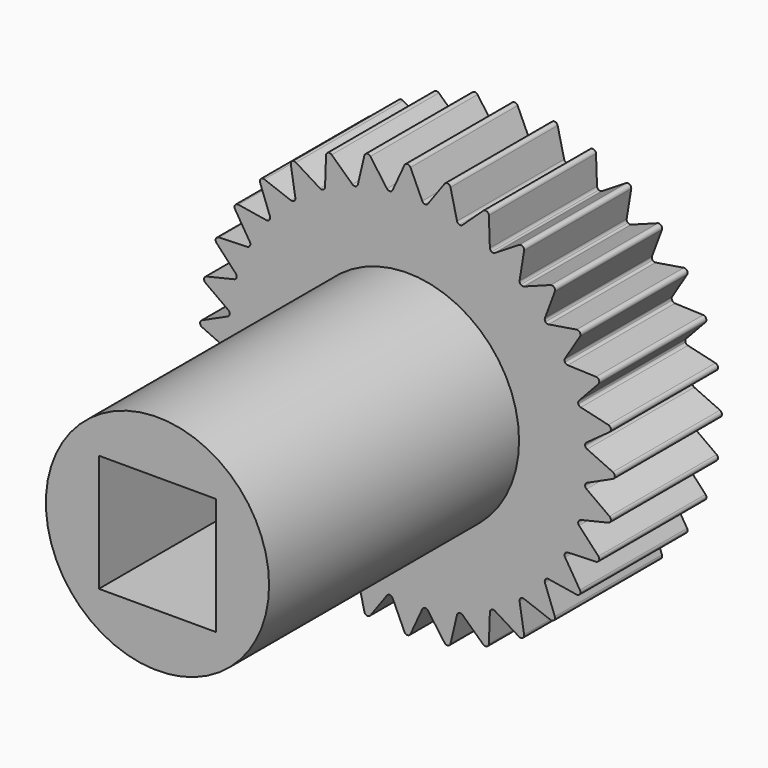
from build123d import *

# Parameters (mm, degrees)
F0_R            = 8
F0_R_2          = 5
F1_DEPTH        = 6
F2_DEPTH        = 20
F3_W            = 5.25
F3_H            = 5.25
F4_DEPTH        = 26
F6_DEPTH        = 6
F6_COPIES_COUNT = 32
F7_T1_DEPTH     = 6
F7_T3_DEPTH     = 7.6415271023


# Not quite as in the source:
# - a fillet or chamfer that OpenCascade refuses, or shapes differently, is made with other operations: its cross-section is extruded or revolved along the edge and cut away or added
# - a pattern or mirror of a feature is missing from the dataset's text; its kind, count and spacing are read off the source's solid


with BuildPart() as f1:
    # F0 (on Front) → F1 (new body)
    with BuildSketch(Plane.XZ):
        Circle(F0_R)
        Circle(F0_R_2, mode=Mode.SUBTRACT)
        Circle(F0_R_2)
    extrude(amount=F1_DEPTH)

    # F0 (on Front) → F2 (join)
    with BuildSketch(Plane.XZ):
        Circle(F0_R_2)
    extrude(amount=F2_DEPTH)

    # F3 (on face) → F4 (cut)
    with BuildSketch(Plane.XZ.offset(20)):
        Rectangle(F3_W, F3_H)
    extrude(amount=-F4_DEPTH, mode=Mode.SUBTRACT)

    # F5 (on face) → F6 (join)
    with BuildSketch(Plane(origin=(0, 0, 0), x_dir=(-1, 0, 0), z_dir=(0, 1, 0))):
        with BuildLine():
            ThreePointArc((-0.6993297572, 7.969375), (-0.35, 7.9923400829), (0, 8))
            ThreePointArc((0, 8), (0.35, 7.9923400829), (0.6993297572, 7.969375))
            Line((0.6993297572, 7.969375), (0, 9.5))
            Line((0, 9.5), (-0.6993297572, 7.969375))
        make_face()
    f6 = extrude(amount=-F6_DEPTH)

    # F6_copies: F6 ×32 about axis
    f6_copies_axis = Axis((0, 0, 0), (0, 1, 0))
    for i in range(1, F6_COPIES_COUNT):
        add(f6.rotate(f6_copies_axis, i * 360 / F6_COPIES_COUNT))

    # F7: fillet of radius 0.15 on 96 edges, made by hand

    # F7_s2 → F7_t1 (join)
    with BuildSketch(Plane.XZ):
        with BuildLine():
            ThreePointArc((0.6632529517, 8.0483364054), (0.7125009612, 7.9886122754), (0.7849689133, 7.9613958453))
            ThreePointArc((0.7849689133, 7.9613958453), (0.7421600586, 7.9655005146), (0.6993297572, 7.969375))
            Line((0.6993297572, 7.969375), (0.6632529517, 8.0483364054))
        make_face()
        with BuildLine():
            ThreePointArc((-0.7849689133, 7.9613958453), (-0.7125009612, 7.9886122754), (-0.6632529517, 8.0483364054))
            Line((-0.6632529517, 8.0483364054), (-0.6993297572, 7.969375))
            ThreePointArc((-0.6993297572, 7.969375), (-0.7421600586, 7.9655005146), (-0.7849689133, 7.9613958453))
        make_face()
        with BuildLine():
            ThreePointArc((-0.7833053234, 7.9615596946), (-0.8596904862, 7.9741153725), (-0.9196438088, 8.0230841101))
            Line((-0.9196438088, 8.0230841101), (-0.868855603, 7.9526781616))
            ThreePointArc((-0.868855603, 7.9526781616), (-0.8260923992, 7.9572339005), (-0.7833053234, 7.9615596946))
        make_face()
        with BuildLine():
            ThreePointArc((-2.3214775758, 7.6557652697), (-2.3988445104, 7.6531776878), (-2.4671991735, 7.6895091918))
            Line((-2.4671991735, 7.6895091918), (-2.4036513296, 7.6303643613))
            ThreePointArc((-2.4036513296, 7.6303643613), (-2.3625985894, 7.6431752502), (-2.3214775758, 7.6557652697))
        make_face()
        with BuildLine():
            ThreePointArc((-2.3230772349, 7.6552800184), (-2.2573113963, 7.6961112886), (-2.2206612733, 7.7642956462))
            Line((-2.2206612733, 7.7642956462), (-2.2406402671, 7.6798132265))
            ThreePointArc((-2.2406402671, 7.6798132265), (-2.2818917216, 7.6676574109), (-2.3230772349, 7.6552800184))
        make_face()
        with BuildLine():
            ThreePointArc((-3.6927308274, 7.1818773596), (-3.7153746204, 7.107853061), (-3.7719110012, 7.0549760736))
            ThreePointArc((-3.7719110012, 7.0549760736), (-3.7339315654, 7.075150533), (-3.695844228, 7.0951205375))
            Line((-3.695844228, 7.0951205375), (-3.6927308274, 7.1818773596))
        make_face()
        with BuildLine():
            ThreePointArc((-3.7704367469, 7.0557640789), (-3.8458122853, 7.0381326765), (-3.9199414575, 7.0604307476))
            Line((-3.9199414575, 7.0604307476), (-3.8460760836, 7.0148199377))
            ThreePointArc((-3.8460760836, 7.0148199377), (-3.8083114408, 7.0353936613), (-3.7704367469, 7.0557640789))
        make_face()
        with BuildLine():
            ThreePointArc((-5.0228908068, 6.3234635537), (-5.0306580813, 6.2464440264), (-5.0757923429, 6.1835533548))
            ThreePointArc((-5.0757923429, 6.1835533548), (-5.0424785132, 6.2107495879), (-5.0090189679, 6.2377663454))
            Line((-5.0090189679, 6.2377663454), (-5.0228908068, 6.3234635537))
        make_face()
        with BuildLine():
            ThreePointArc((-5.0745001483, 6.1846138315), (-5.1449876509, 6.1526161735), (-5.2220425897, 6.1600239093))
            Line((-5.2220425897, 6.1600239093), (-5.1406982907, 6.129699918))
            ThreePointArc((-5.1406982907, 6.129699918), (-5.1076730192, 6.1572458396), (-5.0745001483, 6.1846138315))
        make_face()
        with BuildLine():
            ThreePointArc((-6.1600239093, 5.2220425897), (-6.1526161735, 5.1449876509), (-6.1846138315, 5.0745001483))
            ThreePointArc((-6.1846138315, 5.0745001483), (-6.1572458396, 5.1076730192), (-6.129699918, 5.1406982907))
            Line((-6.129699918, 5.1406982907), (-6.1600239093, 5.2220425897))
        make_face()
        with BuildLine():
            ThreePointArc((-6.1835533548, 5.0757923429), (-6.2464440264, 5.0306580813), (-6.3234635537, 5.0228908068))
            Line((-6.3234635537, 5.0228908068), (-6.2377663454, 5.0090189679))
            ThreePointArc((-6.2377663454, 5.0090189679), (-6.2107495879, 5.0424785132), (-6.1835533548, 5.0757923429))
        make_face()
        with BuildLine():
            ThreePointArc((-7.0604307476, 3.9199414575), (-7.0381326765, 3.8458122853), (-7.0557640789, 3.7704367469))
            ThreePointArc((-7.0557640789, 3.7704367469), (-7.0353936613, 3.8083114408), (-7.0148199377, 3.8460760836))
            Line((-7.0148199377, 3.8460760836), (-7.0604307476, 3.9199414575))
        make_face()
        with BuildLine():
            ThreePointArc((-7.0549760736, 3.7719110012), (-7.107853061, 3.7153746204), (-7.1818773596, 3.6927308274))
            Line((-7.1818773596, 3.6927308274), (-7.0951205375, 3.695844228))
            ThreePointArc((-7.0951205375, 3.695844228), (-7.075150533, 3.7339315654), (-7.0549760736, 3.7719110012))
        make_face()
        with BuildLine():
            ThreePointArc((-7.6895091918, 2.4671991735), (-7.6531776878, 2.3988445104), (-7.6557652697, 2.3214775758))
            ThreePointArc((-7.6557652697, 2.3214775758), (-7.6431752502, 2.3625985894), (-7.6303643613, 2.4036513296))
            Line((-7.6303643613, 2.4036513296), (-7.6895091918, 2.4671991735))
        make_face()
        with BuildLine():
            ThreePointArc((-7.6552800184, 2.3230772349), (-7.6961112886, 2.2573113963), (-7.7642956462, 2.2206612733))
            Line((-7.7642956462, 2.2206612733), (-7.6798132265, 2.2406402671))
            ThreePointArc((-7.6798132265, 2.2406402671), (-7.6676574109, 2.2818917216), (-7.6552800184, 2.3230772349))
        make_face()
        with BuildLine():
            ThreePointArc((-8.0230841101, 0.9196438088), (-7.9741153725, 0.8596904862), (-7.9615596946, 0.7833053234))
            ThreePointArc((-7.9615596946, 0.7833053234), (-7.9572339005, 0.8260923992), (-7.9526781616, 0.868855603))
            Line((-7.9526781616, 0.868855603), (-8.0230841101, 0.9196438088))
        make_face()
        with BuildLine():
            ThreePointArc((-7.9613958453, 0.7849689133), (-7.9886122754, 0.7125009612), (-8.0483364054, 0.6632529517))
            Line((-8.0483364054, 0.6632529517), (-7.969375, 0.6993297572))
            ThreePointArc((-7.969375, 0.6993297572), (-7.9655005146, 0.7421600586), (-7.9613958453, 0.7849689133))
        make_face()
        with BuildLine():
            ThreePointArc((-8.0483364054, -0.6632529517), (-7.9886122754, -0.7125009612), (-7.9613958453, -0.7849689133))
            ThreePointArc((-7.9613958453, -0.7849689133), (-7.9655005146, -0.7421600586), (-7.969375, -0.6993297572))
            Line((-7.969375, -0.6993297572), (-8.0483364054, -0.6632529517))
        make_face()
        with BuildLine():
            ThreePointArc((-7.9615596946, -0.7833053234), (-7.9741153725, -0.8596904862), (-8.0230841101, -0.9196438088))
            Line((-8.0230841101, -0.9196438088), (-7.9526781616, -0.868855603))
            ThreePointArc((-7.9526781616, -0.868855603), (-7.9572339005, -0.8260923992), (-7.9615596946, -0.7833053234))
        make_face()
        with BuildLine():
            ThreePointArc((-7.7642956462, -2.2206612733), (-7.6961112886, -2.2573113963), (-7.6552800184, -2.3230772349))
            ThreePointArc((-7.6552800184, -2.3230772349), (-7.6676574109, -2.2818917216), (-7.6798132265, -2.2406402671))
            Line((-7.6798132265, -2.2406402671), (-7.7642956462, -2.2206612733))
        make_face()
        with BuildLine():
            ThreePointArc((-7.6557652697, -2.3214775758), (-7.6531776878, -2.3988445104), (-7.6895091918, -2.4671991735))
            Line((-7.6895091918, -2.4671991735), (-7.6303643613, -2.4036513296))
            ThreePointArc((-7.6303643613, -2.4036513296), (-7.6431752502, -2.3625985894), (-7.6557652697, -2.3214775758))
        make_face()
        with BuildLine():
            ThreePointArc((-7.1818773596, -3.6927308274), (-7.107853061, -3.7153746204), (-7.0549760736, -3.7719110012))
            ThreePointArc((-7.0549760736, -3.7719110012), (-7.075150533, -3.7339315654), (-7.0951205375, -3.695844228))
            Line((-7.0951205375, -3.695844228), (-7.1818773596, -3.6927308274))
        make_face()
        with BuildLine():
            ThreePointArc((-7.0557640789, -3.7704367469), (-7.0381326765, -3.8458122853), (-7.0604307476, -3.9199414575))
            Line((-7.0604307476, -3.9199414575), (-7.0148199377, -3.8460760836))
            ThreePointArc((-7.0148199377, -3.8460760836), (-7.0353936613, -3.8083114408), (-7.0557640789, -3.7704367469))
        make_face()
        with BuildLine():
            ThreePointArc((-6.3234635537, -5.0228908068), (-6.2464440264, -5.0306580813), (-6.1835533548, -5.0757923429))
            ThreePointArc((-6.1835533548, -5.0757923429), (-6.2107495879, -5.0424785132), (-6.2377663454, -5.0090189679))
            Line((-6.2377663454, -5.0090189679), (-6.3234635537, -5.0228908068))
        make_face()
        with BuildLine():
            ThreePointArc((-6.1846138315, -5.0745001483), (-6.1526161735, -5.1449876509), (-6.1600239093, -5.2220425897))
            Line((-6.1600239093, -5.2220425897), (-6.129699918, -5.1406982907))
            ThreePointArc((-6.129699918, -5.1406982907), (-6.1572458396, -5.1076730192), (-6.1846138315, -5.0745001483))
        make_face()
        with BuildLine():
            ThreePointArc((-5.2220425897, -6.1600239093), (-5.1449876509, -6.1526161735), (-5.0745001483, -6.1846138315))
            ThreePointArc((-5.0745001483, -6.1846138315), (-5.1076730192, -6.1572458396), (-5.1406982907, -6.129699918))
            Line((-5.1406982907, -6.129699918), (-5.2220425897, -6.1600239093))
        make_face()
        with BuildLine():
            ThreePointArc((-5.0757923429, -6.1835533548), (-5.0306580813, -6.2464440264), (-5.0228908068, -6.3234635537))
            Line((-5.0228908068, -6.3234635537), (-5.0090189679, -6.2377663454))
            ThreePointArc((-5.0090189679, -6.2377663454), (-5.0424785132, -6.2107495879), (-5.0757923429, -6.1835533548))
        make_face()
        with BuildLine():
            ThreePointArc((-3.9199414575, -7.0604307476), (-3.8458122853, -7.0381326765), (-3.7704367469, -7.0557640789))
            ThreePointArc((-3.7704367469, -7.0557640789), (-3.8083114408, -7.0353936613), (-3.8460760836, -7.0148199377))
            Line((-3.8460760836, -7.0148199377), (-3.9199414575, -7.0604307476))
        make_face()
        with BuildLine():
            ThreePointArc((-3.7719110012, -7.0549760736), (-3.7153746204, -7.107853061), (-3.6927308274, -7.1818773596))
            Line((-3.6927308274, -7.1818773596), (-3.695844228, -7.0951205375))
            ThreePointArc((-3.695844228, -7.0951205375), (-3.7339315654, -7.075150533), (-3.7719110012, -7.0549760736))
        make_face()
        with BuildLine():
            ThreePointArc((-2.4671991735, -7.6895091918), (-2.3988445104, -7.6531776878), (-2.3214775758, -7.6557652697))
            ThreePointArc((-2.3214775758, -7.6557652697), (-2.3625985894, -7.6431752502), (-2.4036513296, -7.6303643613))
            Line((-2.4036513296, -7.6303643613), (-2.4671991735, -7.6895091918))
        make_face()
        with BuildLine():
            ThreePointArc((-2.3230772349, -7.6552800184), (-2.2573113963, -7.6961112886), (-2.2206612733, -7.7642956462))
            Line((-2.2206612733, -7.7642956462), (-2.2406402671, -7.6798132265))
            ThreePointArc((-2.2406402671, -7.6798132265), (-2.2818917216, -7.6676574109), (-2.3230772349, -7.6552800184))
        make_face()
        with BuildLine():
            ThreePointArc((-0.9196438088, -8.0230841101), (-0.8596904862, -7.9741153725), (-0.7833053234, -7.9615596946))
            ThreePointArc((-0.7833053234, -7.9615596946), (-0.8260923992, -7.9572339005), (-0.868855603, -7.9526781616))
            Line((-0.868855603, -7.9526781616), (-0.9196438088, -8.0230841101))
        make_face()
        with BuildLine():
            ThreePointArc((-0.7849689133, -7.9613958453), (-0.7125009612, -7.9886122754), (-0.6632529517, -8.0483364054))
            Line((-0.6632529517, -8.0483364054), (-0.6993297572, -7.969375))
            ThreePointArc((-0.6993297572, -7.969375), (-0.7421600586, -7.9655005146), (-0.7849689133, -7.9613958453))
        make_face()
        with BuildLine():
            ThreePointArc((0.6632529517, -8.0483364054), (0.7125009612, -7.9886122754), (0.7849689133, -7.9613958453))
            ThreePointArc((0.7849689133, -7.9613958453), (0.7421600586, -7.9655005146), (0.6993297572, -7.969375))
            Line((0.6993297572, -7.969375), (0.6632529517, -8.0483364054))
        make_face()
        with BuildLine():
            ThreePointArc((0.7833053234, -7.9615596946), (0.8596904862, -7.9741153725), (0.9196438088, -8.0230841101))
            Line((0.9196438088, -8.0230841101), (0.868855603, -7.9526781616))
            ThreePointArc((0.868855603, -7.9526781616), (0.8260923992, -7.9572339005), (0.7833053234, -7.9615596946))
        make_face()
        with BuildLine():
            ThreePointArc((2.2206612733, -7.7642956462), (2.2573113963, -7.6961112886), (2.3230772349, -7.6552800184))
            ThreePointArc((2.3230772349, -7.6552800184), (2.2818917216, -7.6676574109), (2.2406402671, -7.6798132265))
            Line((2.2406402671, -7.6798132265), (2.2206612733, -7.7642956462))
        make_face()
        with BuildLine():
            ThreePointArc((2.3214775758, -7.6557652697), (2.3988445104, -7.6531776878), (2.4671991735, -7.6895091918))
            Line((2.4671991735, -7.6895091918), (2.4036513296, -7.6303643613))
            ThreePointArc((2.4036513296, -7.6303643613), (2.3625985894, -7.6431752502), (2.3214775758, -7.6557652697))
        make_face()
        with BuildLine():
            ThreePointArc((3.6927308274, -7.1818773596), (3.7153746204, -7.107853061), (3.7719110012, -7.0549760736))
            ThreePointArc((3.7719110012, -7.0549760736), (3.7339315654, -7.075150533), (3.695844228, -7.0951205375))
            Line((3.695844228, -7.0951205375), (3.6927308274, -7.1818773596))
        make_face()
        with BuildLine():
            ThreePointArc((3.7704367469, -7.0557640789), (3.8458122853, -7.0381326765), (3.9199414575, -7.0604307476))
            Line((3.9199414575, -7.0604307476), (3.8460760836, -7.0148199377))
            ThreePointArc((3.8460760836, -7.0148199377), (3.8083114408, -7.0353936613), (3.7704367469, -7.0557640789))
        make_face()
        with BuildLine():
            ThreePointArc((5.0228908068, -6.3234635537), (5.0306580813, -6.2464440264), (5.0757923429, -6.1835533548))
            ThreePointArc((5.0757923429, -6.1835533548), (5.0424785132, -6.2107495879), (5.0090189679, -6.2377663454))
            Line((5.0090189679, -6.2377663454), (5.0228908068, -6.3234635537))
        make_face()
        with BuildLine():
            ThreePointArc((5.0745001483, -6.1846138315), (5.1449876509, -6.1526161735), (5.2220425897, -6.1600239093))
            Line((5.2220425897, -6.1600239093), (5.1406982907, -6.129699918))
            ThreePointArc((5.1406982907, -6.129699918), (5.1076730192, -6.1572458396), (5.0745001483, -6.1846138315))
        make_face()
        with BuildLine():
            ThreePointArc((6.1600239093, -5.2220425897), (6.1526161735, -5.1449876509), (6.1846138315, -5.0745001483))
            ThreePointArc((6.1846138315, -5.0745001483), (6.1572458396, -5.1076730192), (6.129699918, -5.1406982907))
            Line((6.129699918, -5.1406982907), (6.1600239093, -5.2220425897))
        make_face()
        with BuildLine():
            ThreePointArc((6.1835533548, -5.0757923429), (6.2464440264, -5.0306580813), (6.3234635537, -5.0228908068))
            Line((6.3234635537, -5.0228908068), (6.2377663454, -5.0090189679))
            ThreePointArc((6.2377663454, -5.0090189679), (6.2107495879, -5.0424785132), (6.1835533548, -5.0757923429))
        make_face()
        with BuildLine():
            ThreePointArc((7.0604307476, -3.9199414575), (7.0381326765, -3.8458122853), (7.0557640789, -3.7704367469))
            ThreePointArc((7.0557640789, -3.7704367469), (7.0353936613, -3.8083114408), (7.0148199377, -3.8460760836))
            Line((7.0148199377, -3.8460760836), (7.0604307476, -3.9199414575))
        make_face()
        with BuildLine():
            ThreePointArc((7.0549760736, -3.7719110012), (7.107853061, -3.7153746204), (7.1818773596, -3.6927308274))
            Line((7.1818773596, -3.6927308274), (7.0951205375, -3.695844228))
            ThreePointArc((7.0951205375, -3.695844228), (7.075150533, -3.7339315654), (7.0549760736, -3.7719110012))
        make_face()
        with BuildLine():
            ThreePointArc((7.6895091918, -2.4671991735), (7.6531776878, -2.3988445104), (7.6557652697, -2.3214775758))
            ThreePointArc((7.6557652697, -2.3214775758), (7.6431752502, -2.3625985894), (7.6303643613, -2.4036513296))
            Line((7.6303643613, -2.4036513296), (7.6895091918, -2.4671991735))
        make_face()
        with BuildLine():
            ThreePointArc((7.6552800184, -2.3230772349), (7.6961112886, -2.2573113963), (7.7642956462, -2.2206612733))
            Line((7.7642956462, -2.2206612733), (7.6798132265, -2.2406402671))
            ThreePointArc((7.6798132265, -2.2406402671), (7.6676574109, -2.2818917216), (7.6552800184, -2.3230772349))
        make_face()
        with BuildLine():
            ThreePointArc((8.0230841101, -0.9196438088), (7.9741153725, -0.8596904862), (7.9615596946, -0.7833053234))
            ThreePointArc((7.9615596946, -0.7833053234), (7.9572339005, -0.8260923992), (7.9526781616, -0.868855603))
            Line((7.9526781616, -0.868855603), (8.0230841101, -0.9196438088))
        make_face()
        with BuildLine():
            ThreePointArc((7.9613958453, -0.7849689133), (7.9886122754, -0.7125009612), (8.0483364054, -0.6632529517))
            Line((8.0483364054, -0.6632529517), (7.969375, -0.6993297572))
            ThreePointArc((7.969375, -0.6993297572), (7.9655005146, -0.7421600586), (7.9613958453, -0.7849689133))
        make_face()
        with BuildLine():
            ThreePointArc((8.0483364054, 0.6632529517), (7.9886122754, 0.7125009612), (7.9613958453, 0.7849689133))
            ThreePointArc((7.9613958453, 0.7849689133), (7.9655005146, 0.7421600586), (7.969375, 0.6993297572))
            Line((7.969375, 0.6993297572), (8.0483364054, 0.6632529517))
        make_face()
        with BuildLine():
            ThreePointArc((7.9615596946, 0.7833053234), (7.9741153725, 0.8596904862), (8.0230841101, 0.9196438088))
            Line((8.0230841101, 0.9196438088), (7.9526781616, 0.868855603))
            ThreePointArc((7.9526781616, 0.868855603), (7.9572339005, 0.8260923992), (7.9615596946, 0.7833053234))
        make_face()
        with BuildLine():
            ThreePointArc((7.7642956462, 2.2206612733), (7.6961112886, 2.2573113963), (7.6552800184, 2.3230772349))
            ThreePointArc((7.6552800184, 2.3230772349), (7.6676574109, 2.2818917216), (7.6798132265, 2.2406402671))
            Line((7.6798132265, 2.2406402671), (7.7642956462, 2.2206612733))
        make_face()
        with BuildLine():
            ThreePointArc((7.6557652697, 2.3214775758), (7.6531776878, 2.3988445104), (7.6895091918, 2.4671991735))
            Line((7.6895091918, 2.4671991735), (7.6303643613, 2.4036513296))
            ThreePointArc((7.6303643613, 2.4036513296), (7.6431752502, 2.3625985894), (7.6557652697, 2.3214775758))
        make_face()
        with BuildLine():
            ThreePointArc((7.1818773596, 3.6927308274), (7.107853061, 3.7153746204), (7.0549760736, 3.7719110012))
            ThreePointArc((7.0549760736, 3.7719110012), (7.075150533, 3.7339315654), (7.0951205375, 3.695844228))
            Line((7.0951205375, 3.695844228), (7.1818773596, 3.6927308274))
        make_face()
        with BuildLine():
            ThreePointArc((7.0557640789, 3.7704367469), (7.0381326765, 3.8458122853), (7.0604307476, 3.9199414575))
            Line((7.0604307476, 3.9199414575), (7.0148199377, 3.8460760836))
            ThreePointArc((7.0148199377, 3.8460760836), (7.0353936613, 3.8083114408), (7.0557640789, 3.7704367469))
        make_face()
        with BuildLine():
            ThreePointArc((6.3234635537, 5.0228908068), (6.2464440264, 5.0306580813), (6.1835533548, 5.0757923429))
            ThreePointArc((6.1835533548, 5.0757923429), (6.2107495879, 5.0424785132), (6.2377663454, 5.0090189679))
            Line((6.2377663454, 5.0090189679), (6.3234635537, 5.0228908068))
        make_face()
        with BuildLine():
            ThreePointArc((6.1846138315, 5.0745001483), (6.1526161735, 5.1449876509), (6.1600239093, 5.2220425897))
            Line((6.1600239093, 5.2220425897), (6.129699918, 5.1406982907))
            ThreePointArc((6.129699918, 5.1406982907), (6.1572458396, 5.1076730192), (6.1846138315, 5.0745001483))
        make_face()
        with BuildLine():
            ThreePointArc((5.2220425897, 6.1600239093), (5.1449876509, 6.1526161735), (5.0745001483, 6.1846138315))
            ThreePointArc((5.0745001483, 6.1846138315), (5.1076730192, 6.1572458396), (5.1406982907, 6.129699918))
            Line((5.1406982907, 6.129699918), (5.2220425897, 6.1600239093))
        make_face()
        with BuildLine():
            ThreePointArc((5.0757923429, 6.1835533548), (5.0306580813, 6.2464440264), (5.0228908068, 6.3234635537))
            Line((5.0228908068, 6.3234635537), (5.0090189679, 6.2377663454))
            ThreePointArc((5.0090189679, 6.2377663454), (5.0424785132, 6.2107495879), (5.0757923429, 6.1835533548))
        make_face()
        with BuildLine():
            ThreePointArc((3.9199414575, 7.0604307476), (3.8458122853, 7.0381326765), (3.7704367469, 7.0557640789))
            ThreePointArc((3.7704367469, 7.0557640789), (3.8083114408, 7.0353936613), (3.8460760836, 7.0148199377))
            Line((3.8460760836, 7.0148199377), (3.9199414575, 7.0604307476))
        make_face()
        with BuildLine():
            ThreePointArc((3.7719110012, 7.0549760736), (3.7153746204, 7.107853061), (3.6927308274, 7.1818773596))
            Line((3.6927308274, 7.1818773596), (3.695844228, 7.0951205375))
            ThreePointArc((3.695844228, 7.0951205375), (3.7339315654, 7.075150533), (3.7719110012, 7.0549760736))
        make_face()
        with BuildLine():
            ThreePointArc((2.4671991735, 7.6895091918), (2.3988445104, 7.6531776878), (2.3214775758, 7.6557652697))
            ThreePointArc((2.3214775758, 7.6557652697), (2.3625985894, 7.6431752502), (2.4036513296, 7.6303643613))
            Line((2.4036513296, 7.6303643613), (2.4671991735, 7.6895091918))
        make_face()
        with BuildLine():
            ThreePointArc((2.3230772349, 7.6552800184), (2.2573113963, 7.6961112886), (2.2206612733, 7.7642956462))
            Line((2.2206612733, 7.7642956462), (2.2406402671, 7.6798132265))
            ThreePointArc((2.2406402671, 7.6798132265), (2.2818917216, 7.6676574109), (2.3230772349, 7.6552800184))
        make_face()
        with BuildLine():
            ThreePointArc((0.9196438088, 8.0230841101), (0.8596904862, 7.9741153725), (0.7833053234, 7.9615596946))
            ThreePointArc((0.7833053234, 7.9615596946), (0.8260923992, 7.9572339005), (0.868855603, 7.9526781616))
            Line((0.868855603, 7.9526781616), (0.9196438088, 8.0230841101))
        make_face()
    extrude(amount=F7_T1_DEPTH)

    # F7_s4 → F7_t3 (cut)
    with BuildSketch(Plane.XZ.offset(-0.8207635512)):
        with BuildLine():
            ThreePointArc((0.1364341287, 9.20138624), (0, 9.2890506281), (-0.1364341287, 9.20138624))
            Line((-0.1364341287, 9.20138624), (0, 9.5))
            Line((0, 9.5), (0.1364341287, 9.20138624))
        make_face()
        with BuildLine():
            ThreePointArc((-1.6612888194, 9.0512011616), (-1.8122038783, 9.1105641249), (-1.9289139898, 8.9979672054))
            Line((-1.9289139898, 8.9979672054), (-1.8533580592, 9.3174601638))
            Line((-1.8533580592, 9.3174601638), (-1.6612888194, 9.0512011616))
        make_face()
        with BuildLine():
            ThreePointArc((-3.3951693698, 8.5531834986), (-3.5547657778, 8.5819637517), (-3.6472667679, 8.4487613372))
            Line((-3.6472667679, 8.4487613372), (-3.6354926075, 8.7768555589))
            Line((-3.6354926075, 8.7768555589), (-3.3951693698, 8.5531834986))
        make_face()
        with BuildLine():
            ThreePointArc((-4.9985754654, 7.7264717903), (-5.160720022, 7.7235633244), (-5.2254571296, 7.574874309))
            Line((-5.2254571296, 7.574874309), (-5.2779172137, 7.8989613169))
            Line((-5.2779172137, 7.8989613169), (-4.9985754654, 7.7264717903))
        make_face()
        with BuildLine():
            ThreePointArc((-6.4098891091, 6.6028361043), (-6.5683506899, 6.5683506899), (-6.6028361043, 6.4098891091))
            Line((-6.6028361043, 6.4098891091), (-6.7175144213, 6.7175144213))
            Line((-6.7175144213, 6.7175144213), (-6.4098891091, 6.6028361043))
        make_face()
        with BuildLine():
            ThreePointArc((-7.574874309, 5.2254571296), (-7.7235633244, 5.160720022), (-7.7264717903, 4.9985754654))
            Line((-7.7264717903, 4.9985754654), (-7.8989613169, 5.2779172137))
            Line((-7.8989613169, 5.2779172137), (-7.574874309, 5.2254571296))
        make_face()
        with BuildLine():
            ThreePointArc((-8.4487613372, 3.6472667679), (-8.5819637517, 3.5547657778), (-8.5531834986, 3.3951693698))
            Line((-8.5531834986, 3.3951693698), (-8.7768555589, 3.6354926075))
            Line((-8.7768555589, 3.6354926075), (-8.4487613372, 3.6472667679))
        make_face()
        with BuildLine():
            ThreePointArc((-8.9979672054, 1.9289139898), (-9.1105641249, 1.8122038783), (-9.0512011616, 1.6612888194))
            Line((-9.0512011616, 1.6612888194), (-9.3174601638, 1.8533580592))
            Line((-9.3174601638, 1.8533580592), (-8.9979672054, 1.9289139898))
        make_face()
        with BuildLine():
            ThreePointArc((-9.20138624, 0.1364341287), (-9.2890506281, 0), (-9.20138624, -0.1364341287))
            Line((-9.20138624, -0.1364341287), (-9.5, 0))
            Line((-9.5, 0), (-9.20138624, 0.1364341287))
        make_face()
        with BuildLine():
            ThreePointArc((-9.0512011616, -1.6612888194), (-9.1105641249, -1.8122038783), (-8.9979672054, -1.9289139898))
            Line((-8.9979672054, -1.9289139898), (-9.3174601638, -1.8533580592))
            Line((-9.3174601638, -1.8533580592), (-9.0512011616, -1.6612888194))
        make_face()
        with BuildLine():
            ThreePointArc((-8.5531834986, -3.3951693698), (-8.5819637517, -3.5547657778), (-8.4487613372, -3.6472667679))
            Line((-8.4487613372, -3.6472667679), (-8.7768555589, -3.6354926075))
            Line((-8.7768555589, -3.6354926075), (-8.5531834986, -3.3951693698))
        make_face()
        with BuildLine():
            ThreePointArc((-7.7264717903, -4.9985754654), (-7.7235633244, -5.160720022), (-7.574874309, -5.2254571296))
            Line((-7.574874309, -5.2254571296), (-7.8989613169, -5.2779172137))
            Line((-7.8989613169, -5.2779172137), (-7.7264717903, -4.9985754654))
        make_face()
        with BuildLine():
            ThreePointArc((-6.6028361043, -6.4098891091), (-6.5683506899, -6.5683506899), (-6.4098891091, -6.6028361043))
            Line((-6.4098891091, -6.6028361043), (-6.7175144213, -6.7175144213))
            Line((-6.7175144213, -6.7175144213), (-6.6028361043, -6.4098891091))
        make_face()
        with BuildLine():
            ThreePointArc((-5.2254571296, -7.574874309), (-5.160720022, -7.7235633244), (-4.9985754654, -7.7264717903))
            Line((-4.9985754654, -7.7264717903), (-5.2779172137, -7.8989613169))
            Line((-5.2779172137, -7.8989613169), (-5.2254571296, -7.574874309))
        make_face()
        with BuildLine():
            ThreePointArc((-3.6472667679, -8.4487613372), (-3.5547657778, -8.5819637517), (-3.3951693698, -8.5531834986))
            Line((-3.3951693698, -8.5531834986), (-3.6354926075, -8.7768555589))
            Line((-3.6354926075, -8.7768555589), (-3.6472667679, -8.4487613372))
        make_face()
        with BuildLine():
            ThreePointArc((-1.9289139898, -8.9979672054), (-1.8122038783, -9.1105641249), (-1.6612888194, -9.0512011616))
            Line((-1.6612888194, -9.0512011616), (-1.8533580592, -9.3174601638))
            Line((-1.8533580592, -9.3174601638), (-1.9289139898, -8.9979672054))
        make_face()
        with BuildLine():
            ThreePointArc((-0.1364341287, -9.20138624), (0, -9.2890506281), (0.1364341287, -9.20138624))
            Line((0.1364341287, -9.20138624), (0, -9.5))
            Line((0, -9.5), (-0.1364341287, -9.20138624))
        make_face()
        with BuildLine():
            ThreePointArc((1.6612888194, -9.0512011616), (1.8122038783, -9.1105641249), (1.9289139898, -8.9979672054))
            Line((1.9289139898, -8.9979672054), (1.8533580592, -9.3174601638))
            Line((1.8533580592, -9.3174601638), (1.6612888194, -9.0512011616))
        make_face()
        with BuildLine():
            ThreePointArc((3.3951693698, -8.5531834986), (3.5547657778, -8.5819637517), (3.6472667679, -8.4487613372))
            Line((3.6472667679, -8.4487613372), (3.6354926075, -8.7768555589))
            Line((3.6354926075, -8.7768555589), (3.3951693698, -8.5531834986))
        make_face()
        with BuildLine():
            ThreePointArc((4.9985754654, -7.7264717903), (5.160720022, -7.7235633244), (5.2254571296, -7.574874309))
            Line((5.2254571296, -7.574874309), (5.2779172137, -7.8989613169))
            Line((5.2779172137, -7.8989613169), (4.9985754654, -7.7264717903))
        make_face()
        with BuildLine():
            ThreePointArc((6.4098891091, -6.6028361043), (6.5683506899, -6.5683506899), (6.6028361043, -6.4098891091))
            Line((6.6028361043, -6.4098891091), (6.7175144213, -6.7175144213))
            Line((6.7175144213, -6.7175144213), (6.4098891091, -6.6028361043))
        make_face()
        with BuildLine():
            ThreePointArc((7.574874309, -5.2254571296), (7.7235633244, -5.160720022), (7.7264717903, -4.9985754654))
            Line((7.7264717903, -4.9985754654), (7.8989613169, -5.2779172137))
            Line((7.8989613169, -5.2779172137), (7.574874309, -5.2254571296))
        make_face()
        with BuildLine():
            ThreePointArc((8.4487613372, -3.6472667679), (8.5819637517, -3.5547657778), (8.5531834986, -3.3951693698))
            Line((8.5531834986, -3.3951693698), (8.7768555589, -3.6354926075))
            Line((8.7768555589, -3.6354926075), (8.4487613372, -3.6472667679))
        make_face()
        with BuildLine():
            ThreePointArc((8.9979672054, -1.9289139898), (9.1105641249, -1.8122038783), (9.0512011616, -1.6612888194))
            Line((9.0512011616, -1.6612888194), (9.3174601638, -1.8533580592))
            Line((9.3174601638, -1.8533580592), (8.9979672054, -1.9289139898))
        make_face()
        with BuildLine():
            ThreePointArc((9.20138624, -0.1364341287), (9.2890506281, 0), (9.20138624, 0.1364341287))
            Line((9.20138624, 0.1364341287), (9.5, 0))
            Line((9.5, 0), (9.20138624, -0.1364341287))
        make_face()
        with BuildLine():
            ThreePointArc((9.0512011616, 1.6612888194), (9.1105641249, 1.8122038783), (8.9979672054, 1.9289139898))
            Line((8.9979672054, 1.9289139898), (9.3174601638, 1.8533580592))
            Line((9.3174601638, 1.8533580592), (9.0512011616, 1.6612888194))
        make_face()
        with BuildLine():
            ThreePointArc((8.5531834986, 3.3951693698), (8.5819637517, 3.5547657778), (8.4487613372, 3.6472667679))
            Line((8.4487613372, 3.6472667679), (8.7768555589, 3.6354926075))
            Line((8.7768555589, 3.6354926075), (8.5531834986, 3.3951693698))
        make_face()
        with BuildLine():
            ThreePointArc((7.7264717903, 4.9985754654), (7.7235633244, 5.160720022), (7.574874309, 5.2254571296))
            Line((7.574874309, 5.2254571296), (7.8989613169, 5.2779172137))
            Line((7.8989613169, 5.2779172137), (7.7264717903, 4.9985754654))
        make_face()
        with BuildLine():
            ThreePointArc((6.6028361043, 6.4098891091), (6.5683506899, 6.5683506899), (6.4098891091, 6.6028361043))
            Line((6.4098891091, 6.6028361043), (6.7175144213, 6.7175144213))
            Line((6.7175144213, 6.7175144213), (6.6028361043, 6.4098891091))
        make_face()
        with BuildLine():
            ThreePointArc((5.2254571296, 7.574874309), (5.160720022, 7.7235633244), (4.9985754654, 7.7264717903))
            Line((4.9985754654, 7.7264717903), (5.2779172137, 7.8989613169))
            Line((5.2779172137, 7.8989613169), (5.2254571296, 7.574874309))
        make_face()
        with BuildLine():
            ThreePointArc((3.6472667679, 8.4487613372), (3.5547657778, 8.5819637517), (3.3951693698, 8.5531834986))
            Line((3.3951693698, 8.5531834986), (3.6354926075, 8.7768555589))
            Line((3.6354926075, 8.7768555589), (3.6472667679, 8.4487613372))
        make_face()
        with BuildLine():
            ThreePointArc((1.9289139898, 8.9979672054), (1.8122038783, 9.1105641249), (1.6612888194, 9.0512011616))
            Line((1.6612888194, 9.0512011616), (1.8533580592, 9.3174601638))
            Line((1.8533580592, 9.3174601638), (1.9289139898, 8.9979672054))
        make_face()
    extrude(amount=F7_T3_DEPTH, mode=Mode.SUBTRACT)


solid = f1.part
